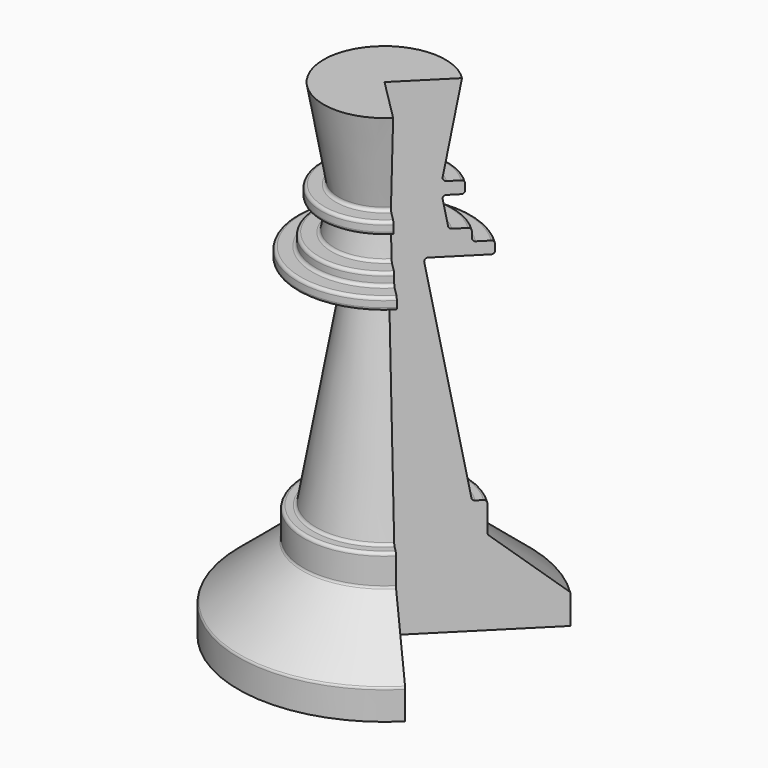
from build123d import *

# Parameters (mm, degrees)
F1_ANGLE_BACK = 135
F1_ANGLE      = 270


# Not quite as in the source:
# - a feature of the source that left no trace in its solid (it failed there, or was rolled back) is left out


with BuildPart() as f1:
    # F0 (on Front) → F1 (revolve)
    with BuildSketch(Plane.XZ, mode=Mode.PRIVATE) as f1_sk:
        with BuildLine():
            Line((-15.24, 0), (0, 0))
            Line((0, 0), (0, 50.8))
            Line((0, 50.8), (-6.35, 50.8))
            Line((-6.35, 50.8), (-4.7617064118, 41.792339449))
            ThreePointArc((-4.7617064118, 41.792339449), (-4.8311637627, 41.5331210865), (-5.0743828734, 41.4197061526))
            Line((-5.0743828734, 41.4197061526), (-6.2835011077, 41.4197061526))
            ThreePointArc((-6.2835011077, 41.4197061526), (-6.5080075107, 41.3267125556), (-6.6010011077, 41.1022061526))
            Line((-6.6010011077, 41.1022061526), (-6.6010011077, 40.4672061526))
            ThreePointArc((-6.6010011077, 40.4672061526), (-6.5080075107, 40.2426997495), (-6.2835011077, 40.1497061526))
            Line((-6.2835011077, 40.1497061526), (-5.0743828734, 40.1497061526))
            ThreePointArc((-5.0743828734, 40.1497061526), (-4.8311637627, 40.0362912186), (-4.7617064118, 39.7770728561))
            Line((-4.7617064118, 39.7770728561), (-5.2010717431, 37.2853082403))
            ThreePointArc((-5.2010717431, 37.2853082403), (-5.3096631386, 37.0972224261), (-5.5137482047, 37.0229415367))
            Line((-5.5137482047, 37.0229415367), (-6.8348340718, 37.0229415367))
            ThreePointArc((-6.8348340718, 37.0229415367), (-7.0593404748, 36.9299479398), (-7.1523340718, 36.7054415367))
            Line((-7.1523340718, 36.7054415367), (-7.1523340718, 36.0704415367))
            ThreePointArc((-7.1523340718, 36.0704415367), (-7.2453276688, 35.8459351337), (-7.4698340718, 35.7529415367))
            Line((-7.4698340718, 35.7529415367), (-8.7398340718, 35.7529415367))
            ThreePointArc((-8.7398340718, 35.7529415367), (-8.9643404748, 35.6599479398), (-9.0573340718, 35.4354415367))
            Line((-9.0573340718, 35.4354415367), (-9.0573340718, 34.8004415367))
            ThreePointArc((-9.0573340718, 34.8004415367), (-8.9643404748, 34.5759351337), (-8.7398340718, 34.4829415367))
            Line((-8.7398340718, 34.4829415367), (-3.5686493249, 34.4829415367))
            ThreePointArc((-3.5686493249, 34.4829415367), (-3.3254302142, 34.3695266028), (-3.2559728633, 34.1103082403))
            Line((-3.2559728633, 34.1103082403), (-7.113602572, 12.2326030065))
            ThreePointArc((-7.113602572, 12.2326030065), (-7.2221939675, 12.0445171922), (-7.4262790336, 11.9702363029))
            Line((-7.4262790336, 11.9702363029), (-8.1123649007, 11.9702363029))
            ThreePointArc((-8.1123649007, 11.9702363029), (-8.3368713037, 11.8772427059), (-8.4298649007, 11.6527363029))
            Line((-8.4298649007, 11.6527363029), (-8.4298649007, 8.9432889844))
            ThreePointArc((-8.4298649007, 8.9432889844), (-8.4596121783, 8.8091076862), (-8.5432798346, 8.7000698737))
            Line((-8.5432798346, 8.7000698737), (-15.1265850661, 3.176020882))
            ThreePointArc((-15.1265850661, 3.176020882), (-15.2102527224, 3.0669830694), (-15.24, 2.9328017713))
            Line((-15.24, 2.9328017713), (-15.24, 0))
        make_face()
    revolve(f1_sk.sketch.rotate(Axis((0, 0, 25.4), (0, 0, 1)), -F1_ANGLE_BACK), axis=Axis((0, 0, 25.4), (0, 0, 1)), revolution_arc=F1_ANGLE)


solid = f1.part
